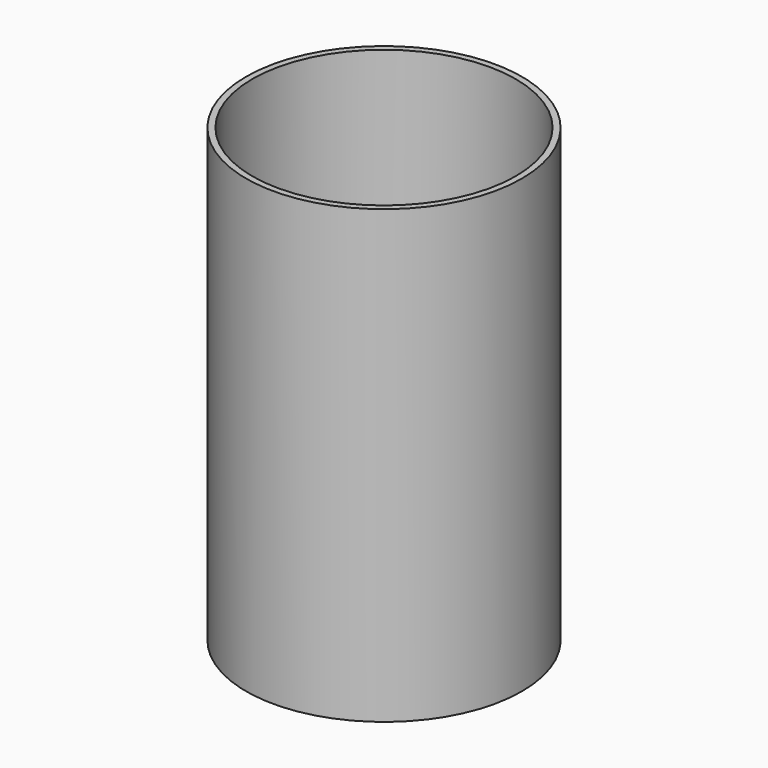
from build123d import *

# Parameters (mm, degrees)
F2_R     = 139.7
F3_DEPTH = 457.2
F4_T     = -6.35


# Not quite as in the source:
# - a variable given as a bare number and used for a length is read in inches; the dataset says mm whatever the document's units were


with BuildPart() as f3:
    # F2 (on Top) → F3 (new body)
    with BuildSketch(Plane.XY):
        Circle(F2_R)
    extrude(amount=F3_DEPTH)

    # F4
    f4_openings = [f3.faces().sort_by_distance(p)[0] for p in [
        (0, 0, 457.2),
    ]]
    offset(amount=F4_T, openings=f4_openings)


solid = f3.part
